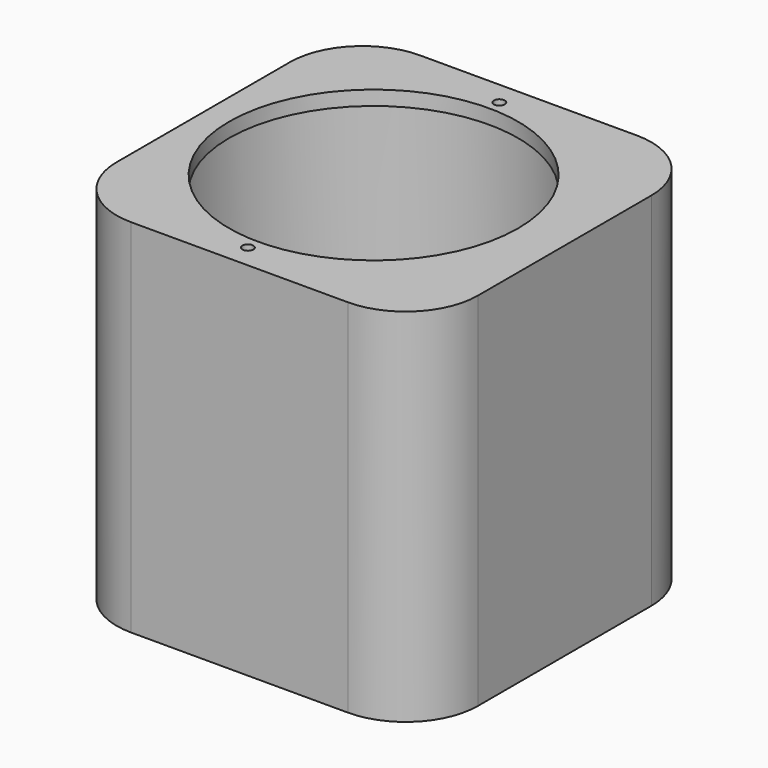
from build123d import *

# Parameters (mm, degrees)
F1_DEPTH  = 50
F2_R      = 20
F3_DEPTH  = 25
F6_R      = 0.75
F7_DEPTH  = 25
F9_DEPTH  = 2
F10_R     = 0.75
F11_DEPTH = 5


# Not quite as in the source:
# - the program builds the solid bodies; features that only make, move or delete a surface that nothing else refers to are left out


with BuildPart() as f1:
    # F0 (on Top) → F1 (new body)
    with BuildSketch(Plane.XY):
        with BuildLine():
            Line((16.436829567, 25), (-13.563170433, 25))
            ThreePointArc((-13.563170433, 25), (-20.6342382449, 22.0710678119), (-23.563170433, 15))
            Line((-23.563170433, 15), (-23.563170433, -15))
            ThreePointArc((-23.563170433, -15), (-20.6342382449, -22.0710678119), (-13.563170433, -25))
            Line((-13.563170433, -25), (16.436829567, -25))
            ThreePointArc((16.436829567, -25), (23.5078973788, -22.0710678119), (26.436829567, -15))
            Line((26.436829567, -15), (26.436829567, 15))
            ThreePointArc((26.436829567, 15), (23.5078973788, 22.0710678119), (16.436829567, 25))
        make_face()
    extrude(amount=F1_DEPTH)

    # F2 (on face) → F3 (cut)
    with BuildSketch(Plane.XY.offset(50)):
        Circle(F2_R)
    extrude(amount=-F3_DEPTH, mode=Mode.SUBTRACT)

    # F4 (on Front) → F5 (revolve, cut)
    with BuildSketch(Plane.XZ):
        Polygon((20, 48), (20, 50), (0, 50), (0, 25), (23, 25), (23, 48), align=None)
    revolve(axis=Axis((0, 0, 37.5), (0, 0, 1)), mode=Mode.SUBTRACT)

    # F6 (on face) → F7 (cut)
    with BuildSketch(Plane.XY.offset(50)):
        with Locations((0, 21.75)):
            Circle(F6_R)
        with Locations((0, -21.75)):
            Circle(F6_R)
    extrude(amount=-F7_DEPTH, mode=Mode.SUBTRACT)

    # F8 (on face) → F9 (cut)
    with BuildSketch(Plane.XY.offset(25)):
        with BuildLine():
            ThreePointArc((7, 4), (6.7071067812, 4.7071067812), (6, 5))
            Line((6, 5), (-6, 5))
            ThreePointArc((-6, 5), (-6.7071067812, 4.7071067812), (-7, 4))
            Line((-7, 4), (-7, -4))
            ThreePointArc((-7, -4), (-6.7071067812, -4.7071067812), (-6, -5))
            Line((-6, -5), (6, -5))
            ThreePointArc((6, -5), (6.7071067812, -4.7071067812), (7, -4))
            Line((7, -4), (7, 4))
        make_face()
    extrude(amount=-F9_DEPTH, mode=Mode.SUBTRACT)

    # F10 (on face) → F11 (cut)
    with BuildSketch(Plane.XY.offset(23)):
        with Locations((-5.4101994716, 3.5321465987)):
            Circle(F10_R)
        with Locations((-5.4101994716, -3.5321465987)):
            Circle(F10_R)
        with Locations((5.4101994716, 3.5321465987)):
            Circle(F10_R)
        with Locations((5.4101994716, -3.5321465987)):
            Circle(F10_R)
    extrude(amount=-F11_DEPTH, mode=Mode.SUBTRACT)


solid = f1.part
